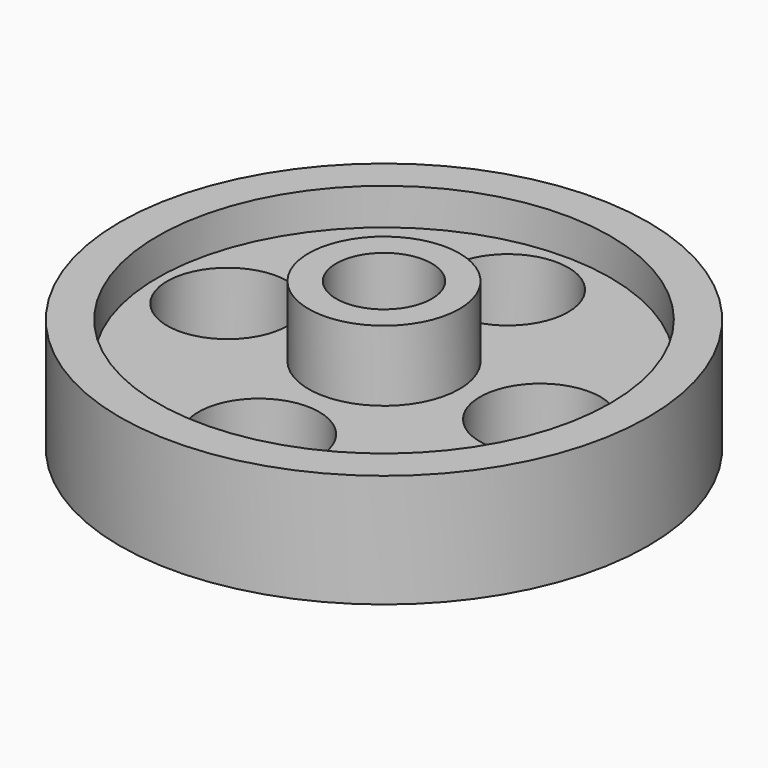
from build123d import *

# Parameters (mm, degrees)
F0_R     = 35.0012
F0_R_2   = 29.9974
F1_DEPTH = 15.0114
F0_R_3   = 8.001
F0_R_4   = 9.9949
F2_DEPTH = 10.16
F0_R_5   = 6.3373
F3_DEPTH = 19.5072


# Not quite as in the source:
# - a feature names something its author has since deleted; it is built from what else it names


with BuildPart() as f1:
    # F0 (on Top) → F1 (new body)
    with BuildSketch(Plane.XY):
        Circle(F0_R)
        Circle(F0_R_2, mode=Mode.SUBTRACT)
    extrude(amount=F1_DEPTH)

    # F0 (on Top) → F2 (join)
    with BuildSketch(Plane.XY):
        Circle(F0_R_2)
        with Locations((0.1067890262, -20.8610873669)):
            Circle(F0_R_3, mode=Mode.SUBTRACT)
        with Locations((20.7458101213, -0.0499814087)):
            Circle(F0_R_3, mode=Mode.SUBTRACT)
        with Locations((-20.7319166511, 0)):
            Circle(F0_R_3, mode=Mode.SUBTRACT)
        Circle(F0_R_4, mode=Mode.SUBTRACT)
        with Locations((0, 20.5026287585)):
            Circle(F0_R_3, mode=Mode.SUBTRACT)
    extrude(amount=F2_DEPTH)

    # F0 (on Top) → F3 (join)
    with BuildSketch(Plane.XY):
        Circle(F0_R_4)
        Circle(F0_R_5, mode=Mode.SUBTRACT)
    extrude(amount=F3_DEPTH)


solid = f1.part
